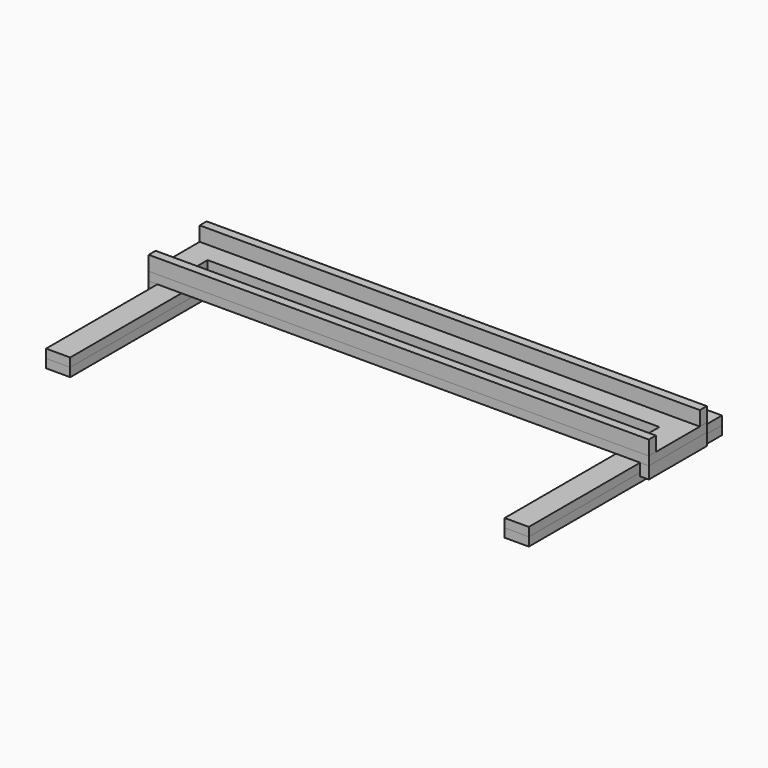
from build123d import *

# Parameters (mm, degrees)
F0_W      = 50
F0_H      = 18
F1_DEPTH  = 500
F2_DEPTH  = 18
F3_W      = 518
F3_H      = 150
F4_DEPTH  = 18
F5_W      = 18
F5_H      = 150
F6_DEPTH  = 25
F9_W      = 1036
F9_H      = 18
F10_DEPTH = 30
F9_W_2    = 936
F9_H_2    = 30
F11_DEPTH = 25


with BuildPart() as f1:
    # F0 (on Front) → F1 (new body)
    with BuildSketch(Plane.XZ):
        with Locations((-27.3853807012, -17.700068422)):
            Rectangle(F0_W, F0_H)
    extrude(amount=F1_DEPTH)


with BuildPart() as f2:
    # F2 (new): a face of the model
    f2_faces = [f1.part.faces().sort_by_distance(p)[0] for p in [
        (-27.3853807012, -250, -8.700068422),
    ]]
    extrude(f2_faces, amount=F2_DEPTH)


with BuildPart() as f4:
    # F3 (on face) → F4 (new body)
    with BuildSketch(Plane.XY.offset(9.299931578)):
        with Locations((188.6146192988, -136.7446185101)):
            Rectangle(F3_W, F3_H)
    extrude(amount=F4_DEPTH)

    # F8: F4 across face


with BuildPart() as f6:
    # F5 (on face) → F6 (new body)
    with BuildSketch(Plane(origin=(0, 0, 9.299931578), x_dir=(1, 0, 0), z_dir=(0, 0, -1))):
        with Locations((-61.3853807012, 136.7446185101)):
            Rectangle(F5_W, F5_H)
    extrude(amount=F6_DEPTH)


with BuildPart() as f7_1:
    # F7: instance of F2
    add(f2.part.mirror(Plane(origin=(447.6146192988, -136.7446185101, 18.299931578), x_dir=(0, 1, 0), z_dir=(1, 0, 0))))


with BuildPart() as f7_2:
    # F7: instance of F1
    add(f1.part.mirror(Plane(origin=(447.6146192988, -136.7446185101, 18.299931578), x_dir=(0, 1, 0), z_dir=(1, 0, 0))))


with BuildPart() as f7_3:
    # F7: instance of F6
    add(f6.part.mirror(Plane(origin=(447.6146192988, -136.7446185101, 18.299931578), x_dir=(0, 1, 0), z_dir=(1, 0, 0))))


with BuildPart() as f4_1:
    add(f4.part)
    add(f4.part.mirror(Plane(origin=(447.6146192988, -136.7446185101, 18.299931578), x_dir=(0, 1, 0), z_dir=(1, 0, 0))))

    # F9 (on face) → F11 (cut)
    with BuildSketch(Plane.XY.offset(27.299931578)):
        with Locations((447.6146192988, -136.7446185101)):
            Rectangle(F9_W_2, F9_H_2)
    extrude(amount=-F11_DEPTH, mode=Mode.SUBTRACT)


with BuildPart() as f10:
    # F9 (on face) → F10 (new body)
    with BuildSketch(Plane.XY.offset(27.299931578)):
        with Locations((447.6146192988, -70.7446185101)):
            Rectangle(F9_W, F9_H)
    extrude(amount=F10_DEPTH)


with BuildPart() as f10b:
    # F9 (on face) → F10, piece 2 (new body)
    with BuildSketch(Plane.XY.offset(27.299931578)):
        with Locations((447.6146192988, -202.7446185101)):
            Rectangle(F9_W, F9_H)
    extrude(amount=F10_DEPTH)


solid = Compound([f1.part, f2.part, f6.part, f7_1.part, f7_2.part, f7_3.part, f4_1.part, f10.part, f10b.part])
